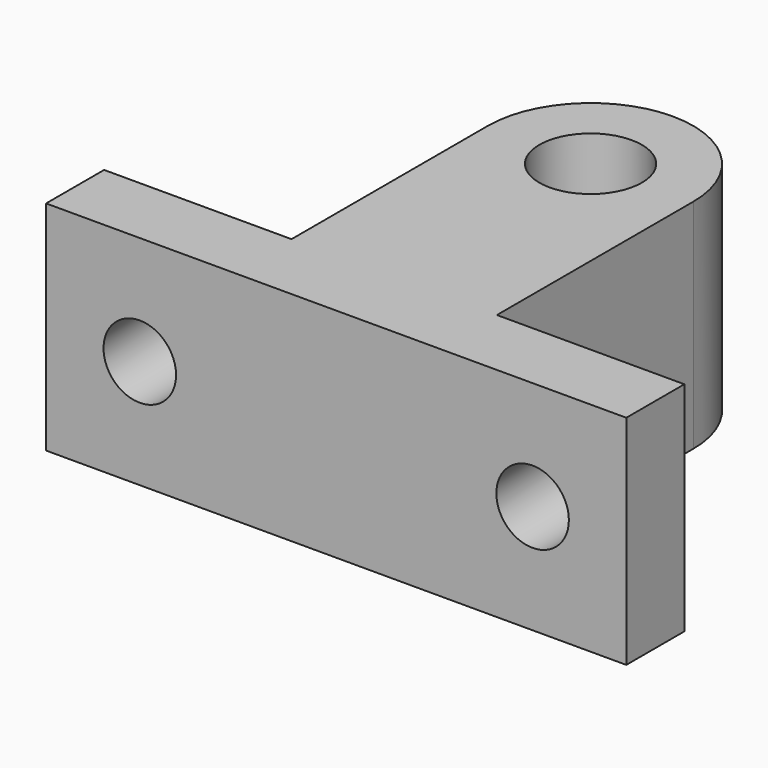
from build123d import *

# Parameters (mm, degrees)
F0_R     = 2.2450679
F1_DEPTH = 9.525
F3_D     = 3.175
F5_D     = 3.175


# Not quite as in the source:
# - a length typed as a fraction of an inch, garbled in the dataset ("3 / 203.2 mm" for 3/8 in), is restored


with BuildPart() as f1:
    # F0 (on Top) → F1 (new body)
    with BuildSketch(Plane.XY):
        with BuildLine():
            Line((14.3843253767, 18.6275094501), (14.3843253767, 7.8833094501))
            Line((14.3843253767, 7.8833094501), (23.3759253767, 7.8833094501))
            Line((23.3759253767, 7.8833094501), (23.3759253767, 18.6275094501))
            ThreePointArc((23.3759253767, 18.6275094501), (22.0591360436, 21.806520117), (18.8801253767, 23.1233094501))
            ThreePointArc((18.8801253767, 23.1233094501), (15.7011147099, 21.806520117), (14.3843253767, 18.6275094501))
        make_face()
        with Locations((18.8801253767, 18.6275094501)):
            Circle(F0_R, mode=Mode.SUBTRACT)
        Polygon((6.1801253767, 7.8833094501), (6.1801253767, 4.7083094501), (31.5801253767, 4.7083094501), (31.5801253767, 7.8833094501), (23.3759253767, 7.8833094501), (14.3843253767, 7.8833094501), align=None)
    extrude(amount=F1_DEPTH)

    # F3 (through all)
    with Locations(Plane(origin=(0, 7.8833094501, 0), x_dir=(-1, 0, 0), z_dir=(0, 1, 0))):
        with Locations((-27.4780253767, 4.7625)):
            Hole(F3_D / 2)

    # F5 (through all)
    with Locations(Plane(origin=(0, 7.8833094501, 0), x_dir=(-1, 0, 0), z_dir=(0, 1, 0))):
        with Locations((-10.2822253767, 4.7625)):
            Hole(F5_D / 2)


solid = f1.part
